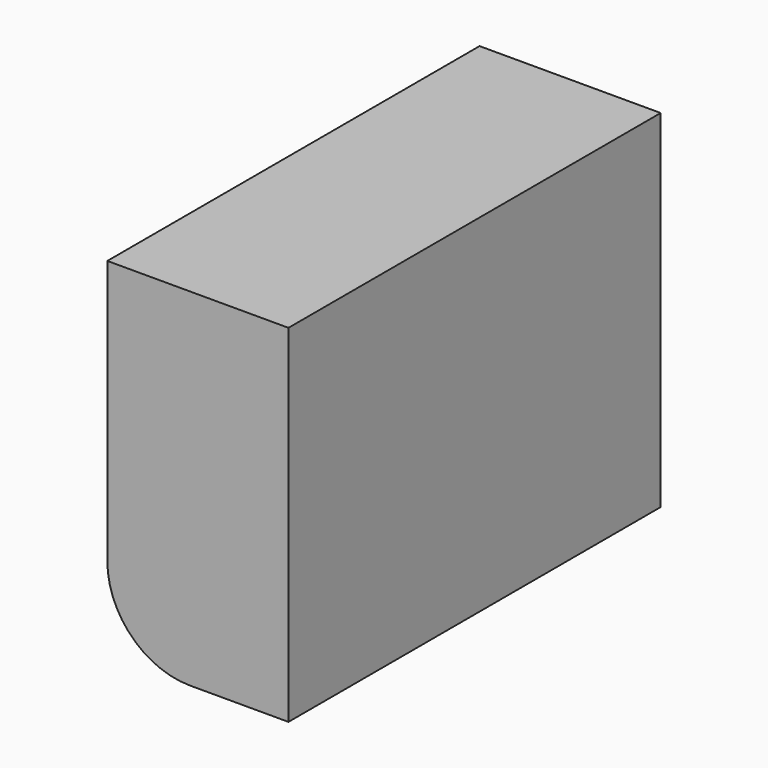
from build123d import *

# Parameters (mm, degrees)
F0_W     = 27.8132706881
F0_H     = 53.2805174589
F1_DEPTH = 71.4483186603
F2_R     = 12.7


# Not quite as in the source:
# - the program builds the solid bodies; features that only make, move or delete a surface that nothing else refers to are left out


with BuildPart() as f1:
    # F0 (on Front) → F1 (new body)
    with BuildSketch(Plane.XZ):
        with Locations((-56.8034946918, -33.0673083663)):
            Rectangle(F0_W, F0_H)
    extrude(amount=F1_DEPTH)

    # F2
    f2_edges = [f1.edges().sort_by_distance(p)[0] for p in [
        (-70.71013, -35.724159, -59.707567),
    ]]
    fillet(f2_edges, radius=F2_R)


solid = f1.part
